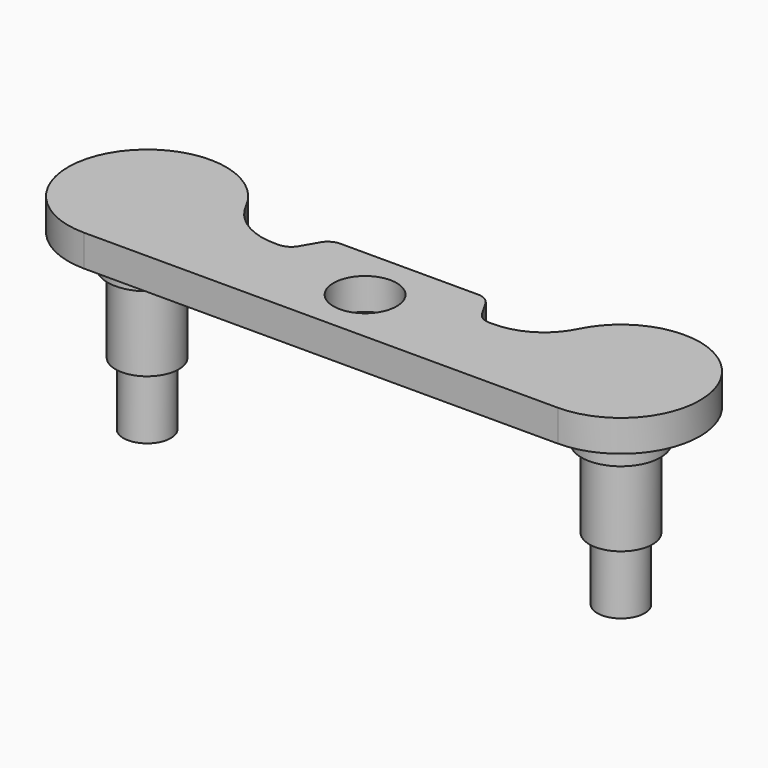
from build123d import *

# Parameters (mm, degrees)
F1_DEPTH = 2
F2_R     = 2.5
F3_DEPTH = 2
F4_R     = 2
F5_DEPTH = 7
F6_R     = 1.5
F7_DEPTH = 11
F8_D     = 4


# Not quite as in the source:
# - a feature names something its author has since deleted; it is built from what else it names


with BuildPart() as f1:
    # F0 (on Top) → F1 (new body)
    with BuildSketch(Plane.XY):
        with BuildLine():
            ThreePointArc((4.4790320824, 2.2222222222), (-4.249182928, 2.6352313835), (0, -5))
            Line((0, -5), (30, -5))
            ThreePointArc((30, -5), (34.249182928, 2.6352313835), (25.5209679176, 2.2222222222))
            ThreePointArc((25.5209679176, 2.2222222222), (24.0459273585, 0.6006536576), (21.9377422517, 0))
            Line((21.9377422517, 0), (21.6697930593, 0))
            ThreePointArc((21.6697930593, 0), (21.1697930593, 0.1339745962), (20.8037676555, 0.5))
            Line((20.8037676555, 0.5), (20.2264173863, 1.5))
            ThreePointArc((20.2264173863, 1.5), (19.8603919825, 1.8660254038), (19.3603919825, 2))
            Line((19.3603919825, 2), (10.6396080175, 2))
            ThreePointArc((10.6396080175, 2), (10.1396080175, 1.8660254038), (9.7735826137, 1.5))
            Line((9.7735826137, 1.5), (9.1962323445, 0.5))
            ThreePointArc((9.1962323445, 0.5), (8.8302069407, 0.1339745962), (8.3302069407, 0))
            Line((8.3302069407, 0), (8.0622577483, 0))
            ThreePointArc((8.0622577483, 0), (5.9540726415, 0.6006536576), (4.4790320824, 2.2222222222))
        make_face()
    extrude(amount=F1_DEPTH)

    # F2 (on Top) → F3 (join)
    with BuildSketch(Plane.XY):
        Circle(F2_R)
        with Locations((30, 0)):
            Circle(F2_R)
    extrude(amount=-F3_DEPTH)

    # F4 (on Top) → F5 (join)
    with BuildSketch(Plane.XY):
        Circle(F4_R)
        with Locations((30, 0)):
            Circle(F4_R)
    extrude(amount=-F5_DEPTH)

    # F6 (on Top) → F7 (join)
    with BuildSketch(Plane.XY):
        Circle(F6_R)
        with Locations((30, 0)):
            Circle(F6_R)
    extrude(amount=-F7_DEPTH)

    # F8 (through all)
    with Locations(Plane(origin=(0, 0, 0), x_dir=(1, 0, 0), z_dir=(0, 0, -1))):
        with Locations((15, 1.5)):
            Hole(F8_D / 2)


solid = f1.part
